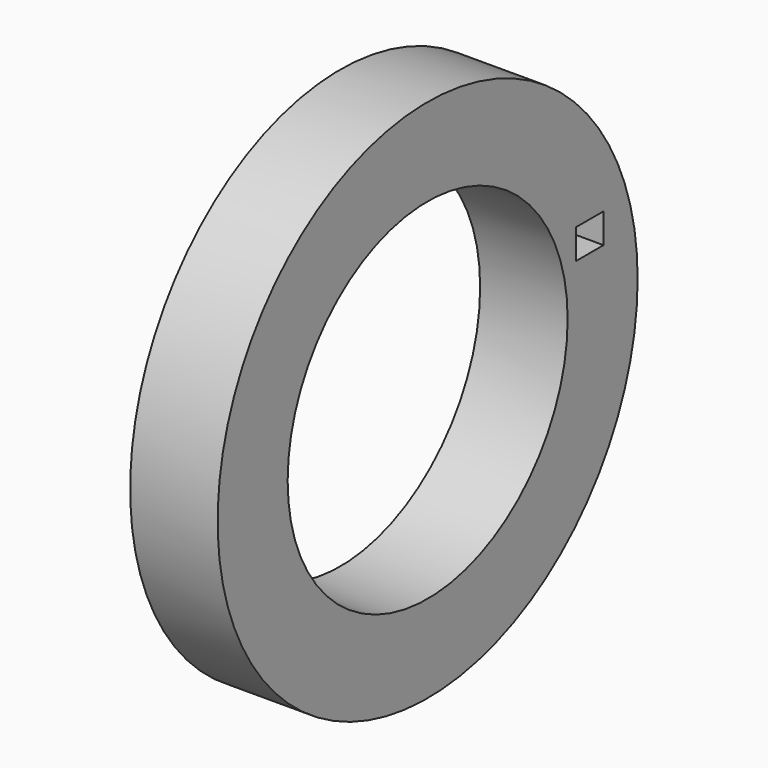
from build123d import *

# Parameters (mm, degrees)
F0_R     = 76.2
F1_DEPTH = 25.4
F2_R     = 50.8
F3_DEPTH = 25.4
F4_W     = 9.9899098277
F4_H     = 8.6538987234
F5_DEPTH = 25.4


# Not quite as in the source:
# - a feature names something its author has since deleted; it is built from what else it names


with BuildPart() as f1:
    # F0 (on Right) → F1 (new body)
    with BuildSketch(Plane.YZ):
        Circle(F0_R)
    extrude(amount=F1_DEPTH)

    # F2 (on face) → F3 (cut)
    with BuildSketch(Plane.YZ.offset(25.4)):
        Circle(F2_R)
    extrude(amount=-F3_DEPTH, mode=Mode.SUBTRACT)

    # F4 (on face) → F5 (cut)
    with BuildSketch(Plane(origin=(0, 0, 0), x_dir=(0, -1, 0), z_dir=(-1, 0, 0))):
        with Locations((-58.8261894882, 17.9770062678)):
            Rectangle(F4_W, F4_H)
    extrude(amount=-F5_DEPTH, mode=Mode.SUBTRACT)


solid = f1.part
